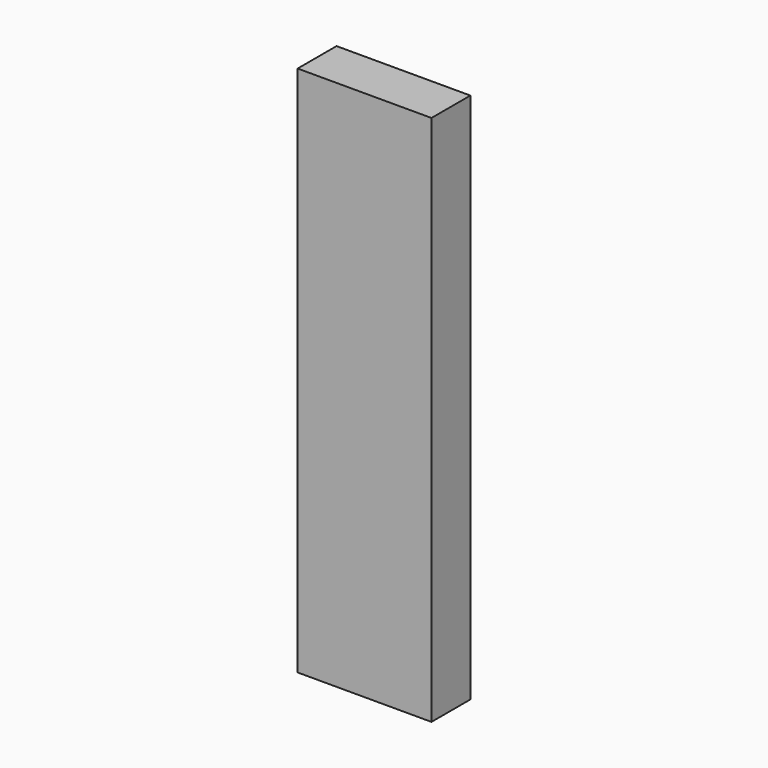
from build123d import *

# Parameters (mm, degrees)
F1_DEPTH = 25.4
F2_DEPTH = 25.4


# Not quite as in the source:
# - the program builds the solid bodies; features that only make, move or delete a surface that nothing else refers to are left out


with BuildPart() as f1:
    # F0 (on Front) → F1 (new body)
    with BuildSketch(Plane.XZ):
        Polygon((34.9633991718, 138.8933360577), (-34.9633991718, 138.8933360577), (-34.9633991718, 40.3722558473), (34.9633991718, 0), align=None)
    extrude(amount=F1_DEPTH)

    # F0 (on Front) → F2 (join)
    with BuildSketch(Plane.XZ):
        Polygon((34.9633991718, 0), (-34.9633991718, 40.3722558473), (-34.9633991718, -138.8933360577), (34.9633991718, -138.8933360577), align=None)
    extrude(amount=F2_DEPTH)


solid = f1.part
